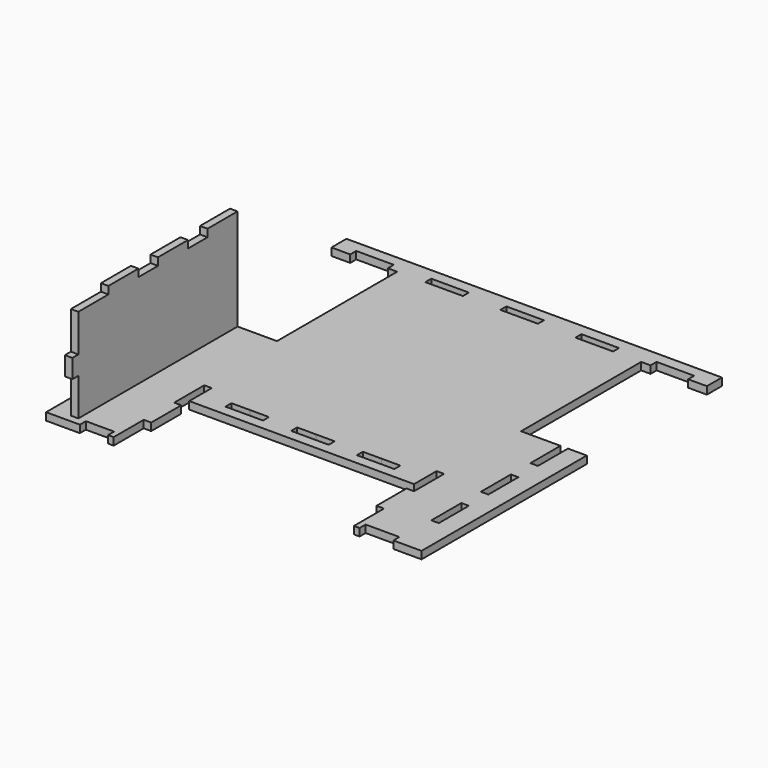
from build123d import *

# Parameters (mm, degrees)
F0_W      = 200
F0_H      = 200
F1_DEPTH  = 4
F2_W      = 4
F2_H      = 20
F3_DEPTH  = 54
F4_W      = 60
F4_H      = 45
F5_DEPTH  = 25
F6_W      = 4
F6_H      = 20
F7_DEPTH  = 4
F11_W     = 4
F11_H     = 176
F12_DEPTH = 50
F13_W     = 70
F13_H     = 23
F14_DEPTH = 4
F15_W     = 4
F15_H     = 5
F16_DEPTH = 4
F17_W     = 15
F17_H     = 4
F18_DEPTH = 4
F19_W     = 4
F19_H     = 20
F20_DEPTH = 4
F21_W     = 18
F21_H     = 4
F21_W_2   = 4
F21_H_2   = 20
F22_DEPTH = 4
F25_DEPTH = 4
F26_W     = 4
F26_H     = 31
F27_DEPTH = 10
F28_W     = 10
F28_H     = 80
F28_W_2   = 25
F29_DEPTH = 25
F30_W     = 80
F30_H     = 31
F31_DEPTH = 25


# Not quite as in the source:
# - ends of sketch curves that miss each other by under 0.0002 mm in the source are joined


with BuildPart() as f1:
    # F0 (on Top) → F1 (new body)
    with BuildSketch(Plane.XY):
        with Locations((-57.977979065, -66.4845939098)):
            Rectangle(F0_W, F0_H)
        Polygon((-143.977979065, -122.4845939098), (-143.977979065, -132.4845939098), (-143.977979065, -142.4845939098), (-147.977979065, -142.4845939098), (-147.977979065, -132.4845939098), (-147.977979065, -122.4845939098), align=None, mode=Mode.SUBTRACT)
        Polygon((-147.977979065, -109.4845939098), (-147.977979065, -99.4845939098), (-147.977979065, -89.4845939098), (-143.977979065, -89.4845939098), (-143.977979065, -99.4845939098), (-143.977979065, -109.4845939098), align=None, mode=Mode.SUBTRACT)
        Polygon((-147.977979065, -66.4845939098), (-147.977979065, -56.4845939098), (-143.977979065, -56.4845939098), (-143.977979065, -66.4845939098), (-143.977979065, -76.4845939098), (-147.977979065, -76.4845939098), align=None, mode=Mode.SUBTRACT)
        Polygon((32.022020935, -122.4845939098), (32.022020935, -132.4845939098), (32.022020935, -142.4845939098), (28.022020935, -142.4845939098), (28.022020935, -132.4845939098), (28.022020935, -122.4845939098), align=None, mode=Mode.SUBTRACT)
        Polygon((32.022020935, -89.4845939098), (32.022020935, -99.4845939098), (32.022020935, -109.4845939098), (28.022020935, -109.4845939098), (28.022020935, -99.4845939098), (28.022020935, -89.4845939098), align=None, mode=Mode.SUBTRACT)
        Polygon((-127.977979065, 23.5154060902), (-137.977979065, 23.5154060902), (-147.977979065, 23.5154060902), (-147.977979065, 27.5154060902), (-137.977979065, 27.5154060902), (-127.977979065, 27.5154060902), align=None, mode=Mode.SUBTRACT)
        Polygon((-87.977979065, 23.5154060902), (-97.977979065, 23.5154060902), (-107.977979065, 23.5154060902), (-107.977979065, 27.5154060902), (-97.977979065, 27.5154060902), (-87.977979065, 27.5154060902), align=None, mode=Mode.SUBTRACT)
        Polygon((32.022020935, -66.4845939098), (32.022020935, -76.4845939098), (28.022020935, -76.4845939098), (28.022020935, -66.4845939098), (28.022020935, -56.4845939098), (32.022020935, -56.4845939098), align=None, mode=Mode.SUBTRACT)
        Polygon((-47.977979065, 23.5154060902), (-57.977979065, 23.5154060902), (-67.977979065, 23.5154060902), (-67.977979065, 27.5154060902), (-57.977979065, 27.5154060902), (-47.977979065, 27.5154060902), align=None, mode=Mode.SUBTRACT)
        Polygon((-7.977979065, 23.5154060902), (-17.977979065, 23.5154060902), (-27.977979065, 23.5154060902), (-27.977979065, 27.5154060902), (-17.977979065, 27.5154060902), (-7.977979065, 27.5154060902), align=None, mode=Mode.SUBTRACT)
        Polygon((32.022020935, 23.5154060902), (22.022020935, 23.5154060902), (12.022020935, 23.5154060902), (12.022020935, 27.5154060902), (22.022020935, 27.5154060902), (32.022020935, 27.5154060902), align=None, mode=Mode.SUBTRACT)
    extrude(amount=F1_DEPTH)

    # F4 (on face) → F5 (cut)
    with BuildSketch(Plane.XY.offset(4)):
        with Locations((-87.977979065, -143.9845939098)):
            Rectangle(F4_W, F4_H)
        with Locations((-27.977979065, -143.9845939098)):
            Rectangle(F4_W, F4_H)
    extrude(amount=-F5_DEPTH, mode=Mode.SUBTRACT)

    # F17 (on face) → F18 (cut)
    with BuildSketch(Plane.XZ.offset(166.4845939098)):
        with Locations((-132.477979065, 2)):
            Rectangle(F17_W, F17_H)
    extrude(amount=-F18_DEPTH, mode=Mode.SUBTRACT)

    # F19 (on face) → F20 (cut)
    with BuildSketch(Plane.XY.offset(4)):
        with Locations((-119.977979065, -156.4845939098)):
            Rectangle(F19_W, F19_H)
        with Locations((-119.7271731991, -116.4853802123)):
            Rectangle(F19_W, F19_H)
    extrude(amount=-F20_DEPTH, mode=Mode.SUBTRACT)

    # F21 (on face) → F22 (cut)
    with BuildSketch(Plane.XY.offset(4)):
        with Locations((18.022020935, -164.4845939098)):
            Rectangle(F21_W, F21_H)
        with Locations((4.022020935, -156.4845939098)):
            Rectangle(F21_W_2, F21_H_2)
        with Locations((4.022020935, -116.4845939098)):
            Rectangle(F21_W_2, F21_H_2)
    extrude(amount=-F22_DEPTH, mode=Mode.SUBTRACT)

    # F24 (on face) → F25 (cut, through all)
    with BuildSketch(Plane.XY.offset(4)):
        Polygon((-47.8525531523, -111.9846591607), (-57.8525531515, -111.9847904856), (-67.8525268865, -111.9847904854), (-67.8525268865, -113.9847904854), (-67.8525268865, -115.9847904854), (-57.8525268865, -115.9847904854), (-47.8525006224, -115.9846591603), (-47.8525268873, -113.9846591605), align=None)
        Polygon((-32.8525268865, -111.9847904854), (-32.8525268865, -113.9847904854), (-32.8525268865, -115.9847904854), (-22.8525268865, -115.9847904854), (-12.8525006224, -115.9846591603), (-12.8525268873, -113.9846591605), (-12.8525531523, -111.9846591607), (-22.8525531515, -111.9847904856), align=None)
        Polygon((-102.8525268865, -115.9847904854), (-92.8525268865, -115.9847904854), (-82.8525006224, -115.9846591603), (-82.8525268873, -113.9846591605), (-82.8525531523, -111.9846591607), (-92.8525531515, -111.9847904856), (-102.8525268865, -111.9847904854), (-102.8525268865, -113.9847904854), align=None)
    extrude(amount=-F25_DEPTH, mode=Mode.SUBTRACT)

    # F28 (on face) → F29 (cut)
    with BuildSketch(Plane(origin=(0, 0, 0), x_dir=(1, 0, 0), z_dir=(0, 0, -1))):
        with Locations((-152.977979065, 16.4845939098)):
            Rectangle(F28_W, F28_H)
        with Locations((-135.477979065, 16.4845939098)):
            Rectangle(F28_W_2, F28_H)
        with Locations((37.022020935, 16.4845939098)):
            Rectangle(F28_W, F28_H)
        with Locations((19.522020935, 16.4845939098)):
            Rectangle(F28_W_2, F28_H)
    extrude(amount=-F29_DEPTH, mode=Mode.SUBTRACT)


with BuildPart() as f3:
    # F2 (on face) → F3 (new body)
    with BuildSketch(Plane.XY.offset(4)):
        with Locations((-145.977979065, -66.4845939098)):
            Rectangle(F2_W, F2_H)
    extrude(amount=F3_DEPTH)

    # F6 (on face) → F7 (join)
    with BuildSketch(Plane(origin=(0, 0, 0), x_dir=(1, 0, 0), z_dir=(0, 0, -1))):
        with Locations((-145.977979065, 66.4845939098)):
            Rectangle(F6_W, F6_H)
    extrude(amount=-F7_DEPTH)

    # F10: union 



with BuildPart() as f3b:
    # F2 (on face) → F3, piece 2 (new body)
    with BuildSketch(Plane.XY.offset(4)):
        with Locations((-145.977979065, -31.4845939098)):
            Rectangle(F2_W, F2_H)
    extrude(amount=F3_DEPTH)


with BuildPart() as f3c:
    # F2 (on face) → F3, piece 3 (new body)
    with BuildSketch(Plane.XY.offset(4)):
        with Locations((-145.977979065, 3.5154060902)):
            Rectangle(F2_W, F2_H)
    extrude(amount=F3_DEPTH)


with BuildPart() as f3d:
    # F2 (on face) → F3, piece 4 (new body)
    with BuildSketch(Plane.XY.offset(4)):
        with Locations((-145.977979065, -99.4845939098)):
            Rectangle(F2_W, F2_H)
    extrude(amount=F3_DEPTH)

    # F6 (on face) → F7, piece 2 (join)
    with BuildSketch(Plane(origin=(0, 0, 0), x_dir=(1, 0, 0), z_dir=(0, 0, -1))):
        with Locations((-145.977979065, 99.4845939098)):
            Rectangle(F6_W, F6_H)
    extrude(amount=-F7_DEPTH)

    # F8: union 


with BuildPart() as f3e:
    # F2 (on face) → F3, piece 5 (new body)
    with BuildSketch(Plane.XY.offset(4)):
        with Locations((-145.977979065, -132.4845939098)):
            Rectangle(F2_W, F2_H)
    extrude(amount=F3_DEPTH)

    # F6 (on face) → F7, piece 3 (join)
    with BuildSketch(Plane(origin=(0, 0, 0), x_dir=(1, 0, 0), z_dir=(0, 0, -1))):
        with Locations((-145.977979065, 132.4845939098)):
            Rectangle(F6_W, F6_H)
    extrude(amount=-F7_DEPTH)

    # F9: union 


with BuildPart() as f3_1:
    add(f3.part)

    add(f3b.part)  # F12 merges F3b

    add(f3c.part)  # F12 merges F3c

    add(f3d.part)  # F12 merges F3d

    add(f3e.part)  # F12 merges F3e
    # F11 (on face) → F12 (join)
    with BuildSketch(Plane.XY.offset(4)):
        with Locations((-145.977979065, -74.4845939098)):
            Rectangle(F11_W, F11_H)
    extrude(amount=F12_DEPTH)

    # F13 (on face) → F14 (cut, through all)
    with BuildSketch(Plane(origin=(-147.977979065, 0, 0), x_dir=(0, -1, 0), z_dir=(-1, 0, 0))):
        with Locations((21.4845939098, 15.5)):
            Rectangle(F13_W, F13_H)
    extrude(amount=-F14_DEPTH, mode=Mode.SUBTRACT)

    # F15 (on face) → F16 (join)
    with BuildSketch(Plane.XZ.offset(162.4845939098)):
        with Locations((-145.977979065, 31.5)):
            Rectangle(F15_W, F15_H)
        with Locations((-145.977979065, 26.5)):
            Rectangle(F15_W, F15_H)
    extrude(amount=F16_DEPTH)

    # F26 (on face) → F27 (join)
    with BuildSketch(Plane(origin=(0, 13.5154060902, 0), x_dir=(-1, 0, 0), z_dir=(0, 1, 0))):
        with Locations((145.977979065, 42.5)):
            Rectangle(F26_W, F26_H)
    extrude(amount=F27_DEPTH)

    # F30 (on face) → F31 (cut)
    with BuildSketch(Plane.YZ.offset(-143.977979065)):
        with Locations((-16.4845939098, 42.5)):
            Rectangle(F30_W, F30_H)
    extrude(amount=-F31_DEPTH, mode=Mode.SUBTRACT)


solid = Compound([f1.part, f3_1.part])
